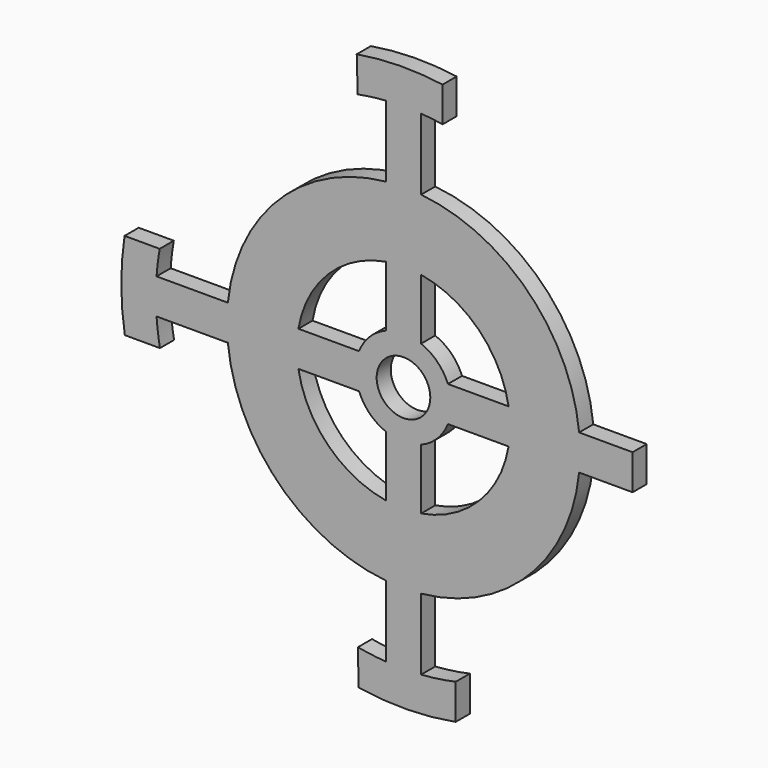
from build123d import *

# Parameters (mm, degrees)
F0_R     = 50.8
F0_R_2   = 4.826
F1_DEPTH = 3.175
F3_DEPTH = 25.4


with BuildPart() as f1:
    # F0 (on Front) → F1 (new body)
    with BuildSketch(Plane.XZ):
        Circle(F0_R)
        with BuildLine():
            Line((-3.175, -31.6174778593), (-3.175, -44.45))
            ThreePointArc((-3.175, -44.45), (-31.5109752705, -31.5109752705), (-44.45, -3.175))
            Line((-44.45, -3.175), (-31.6174778593, -3.175))
            ThreePointArc((-31.6174778593, -3.175), (-22.4693739475, -22.4693739475), (-3.175, -31.6174778593))
        make_face(mode=Mode.SUBTRACT)
        with BuildLine():
            ThreePointArc((-8.001, -3.175), (-6.0867325389, -6.0867325389), (-3.175, -8.001))
            Line((-3.175, -8.001), (-3.175, -18.9174778593))
            ThreePointArc((-3.175, -18.9174778593), (-13.5637677944, -13.5637677944), (-18.9174778593, -3.175))
            Line((-18.9174778593, -3.175), (-8.001, -3.175))
        make_face(mode=Mode.SUBTRACT)
        Circle(F0_R_2, mode=Mode.SUBTRACT)
        with BuildLine():
            Line((31.6174778593, -3.175), (44.45, -3.175))
            ThreePointArc((44.45, -3.175), (31.5109752705, -31.5109752705), (3.175, -44.45))
            Line((3.175, -44.45), (3.175, -31.6174778593))
            ThreePointArc((3.175, -31.6174778593), (22.4693739475, -22.4693739475), (31.6174778593, -3.175))
        make_face(mode=Mode.SUBTRACT)
        with BuildLine():
            ThreePointArc((3.175, -8.001), (6.0867325389, -6.0867325389), (8.001, -3.175))
            Line((8.001, -3.175), (18.9174778593, -3.175))
            ThreePointArc((18.9174778593, -3.175), (13.5637677944, -13.5637677944), (3.175, -18.9174778593))
            Line((3.175, -18.9174778593), (3.175, -8.001))
        make_face(mode=Mode.SUBTRACT)
        with BuildLine():
            Line((-3.175, 18.9174778593), (-3.175, 8.001))
            ThreePointArc((-3.175, 8.001), (-6.0867325389, 6.0867325389), (-8.001, 3.175))
            Line((-8.001, 3.175), (-18.9174778593, 3.175))
            ThreePointArc((-18.9174778593, 3.175), (-13.5637677944, 13.5637677944), (-3.175, 18.9174778593))
        make_face(mode=Mode.SUBTRACT)
        with BuildLine():
            ThreePointArc((-44.45, 3.175), (-31.5109752705, 31.5109752705), (-3.175, 44.45))
            Line((-3.175, 44.45), (-3.175, 37.9674778593))
            Line((-3.175, 37.9674778593), (-3.175, 31.6174778593))
            ThreePointArc((-3.175, 31.6174778593), (-22.4693739475, 22.4693739475), (-31.6174778593, 3.175))
            Line((-31.6174778593, 3.175), (-44.45, 3.175))
        make_face(mode=Mode.SUBTRACT)
        with BuildLine():
            ThreePointArc((8.001, 3.175), (6.0867325389, 6.0867325389), (3.175, 8.001))
            Line((3.175, 8.001), (3.175, 18.9174778593))
            ThreePointArc((3.175, 18.9174778593), (13.5637677944, 13.5637677944), (18.9174778593, 3.175))
            Line((18.9174778593, 3.175), (8.001, 3.175))
        make_face(mode=Mode.SUBTRACT)
        with BuildLine():
            Line((3.175, 37.9674778593), (3.175, 44.45))
            ThreePointArc((3.175, 44.45), (31.5109752705, 31.5109752705), (44.45, 3.175))
            Line((44.45, 3.175), (31.6174778593, 3.175))
            ThreePointArc((31.6174778593, 3.175), (22.4693739475, 22.4693739475), (3.175, 31.6174778593))
            Line((3.175, 31.6174778593), (3.175, 37.9674778593))
        make_face(mode=Mode.SUBTRACT)
    extrude(amount=F1_DEPTH)

    # F2 (on face) → F3 (cut)
    with BuildSketch(Plane.XZ.offset(3.175)):
        Polygon((-39.8937948048, 44.5096977055), (-53.3885769546, 7.7240979299), (-39.592076093, 7.7240979299), (-8.112732321, 39.0091240406), (-8.5013657808, 53.1942620873), align=None)
        Polygon((7.0348572917, 55.979128927), (7.0348572917, 38.4760089219), (40.1488728821, 8.9099211618), (41.2437692285, 8.9099211618), (41.2437692285, 11.4161195233), (53.2457668566, 13.9619985828), (46.2986193597, 36.3472476602), align=None)
        Polygon((41.2437692285, 11.4161195233), (41.2437692285, 8.9099211618), (54.8136532307, 8.9099211618), (53.2457668566, 13.9619985828), align=None)
        Polygon((54.8136532307, 8.9099211618), (41.2437692285, 8.9099211618), (41.2437692285, -6.7063555237), (56.2328249216, -6.7009725608), (55.2191524148, -9.5701087266), (60.481145978, -9.5701087266), (60.481145978, 15.4967764392), (53.2457668566, 13.9619985828), align=None)
        Polygon((41.2437692285, -9.5701087266), (41.2437692285, -6.7063555237), (39.6758913994, -6.7069185898), (9.4001442194, -39.3419340253), (9.4001442194, -54.716296494), (44.45, -40.0515161455), (55.2191524148, -9.5701087266), align=None)
        Polygon((56.2328249216, -6.7009725608), (41.2437692285, -6.7063555237), (41.2437692285, -9.5701087266), (55.2191524148, -9.5701087266), align=None)
        Polygon((-8.001, -54.6349138021), (-8.3070490509, -38.0337389297), (-39.696149528, -8.001), (-54.2215406895, -8.001), (-44.45, -37.7750843763), align=None)
    extrude(amount=-F3_DEPTH, mode=Mode.SUBTRACT)


solid = f1.part
